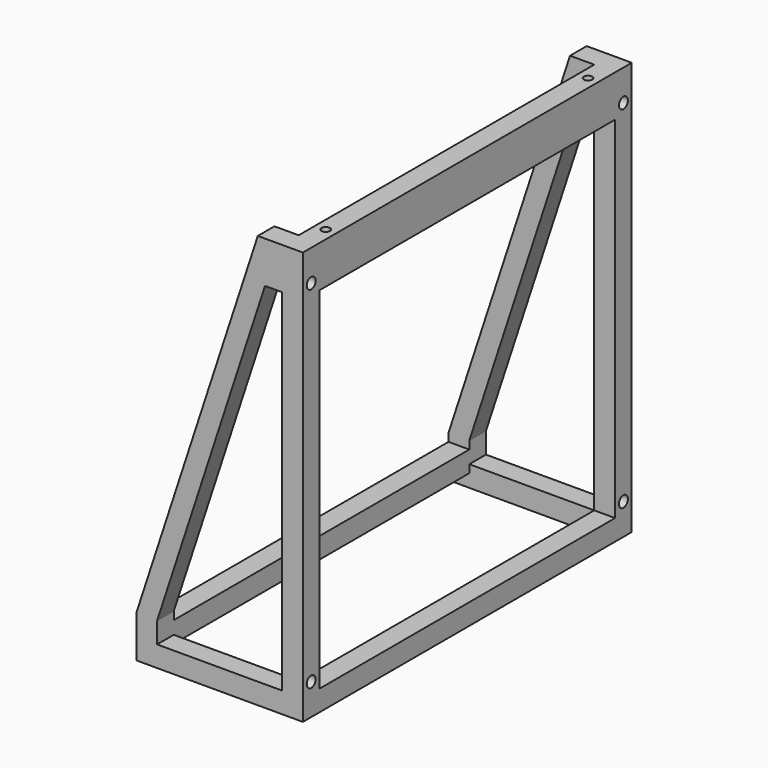
from build123d import *

# Parameters (mm, degrees)
F1_DEPTH = 12.7
F2_W     = 12.7
F2_H     = 12.7
F3_DEPTH = 225.300032
F4_W     = 12.7
F4_H     = 25.4
F5_DEPTH = 12.7
F7_D     = 6.8
F7_DEPTH = 15.75
F7_TIP   = 2.0429261047
F9_D     = 5.1054
F9_DEPTH = 16.51
F9_TIP   = 1.5338169022


# Not quite as in the source:
# - a feature names something its author has since deleted; it is built from what else it names


with BuildPart() as f1:
    # F0 (on Front) → F1 (new body)
    with BuildSketch(Plane.XZ):
        Polygon((0, 25.4), (0, 0), (101.6, 0), (101.6, 226.6), (101.6, 239.3), (101.6, 252), (74.1228589826, 252), align=None)
        Polygon((78.5142949131, 226.6), (88.9, 226.6), (88.9, 12.7), (12.7, 12.7), (12.7, 25.4), align=None, mode=Mode.SUBTRACT)
    extrude(amount=F1_DEPTH)

    # F2 (on face) → F3 (join)
    with BuildSketch(Plane(origin=(0, 0, 0), x_dir=(-1, 0, 0), z_dir=(0, 1, 0))):
        with Locations((-95.25, 6.35)):
            Rectangle(F2_W, F2_H)
        Polygon((-101.6, 252), (-101.6, 226.6), (-88.9, 226.6), (-88.9, 229.1588783264), (-88.9, 252), align=None)
        Polygon((-12.7, 20.574), (-12.7, 12.7), (-12.7, 7.874), (0, 7.874), (0, 20.574), align=None)
    extrude(amount=F3_DEPTH)

    # F4 (on face) → F5 (join)
    with BuildSketch(Plane(origin=(0, 225.300032, 0), x_dir=(-1, 0, 0), z_dir=(0, 1, 0))):
        Polygon((0, 0), (0, 25.4), (-74.1228589826, 252), (-88.9, 252), (-88.9, 226.6), (-101.6, 226.6), (-101.6, 0), align=None)
        Polygon((-88.9, 25.4), (-88.9, 226.6), (-78.5142949131, 226.6), (-12.7, 25.4), (-12.7, 12.7), (-88.9, 12.7), align=None, mode=Mode.SUBTRACT)
        with Locations((-95.25, 239.3)):
            Rectangle(F4_W, F4_H)
    extrude(amount=F5_DEPTH)

    # F7
    with Locations(Plane.YZ.offset(101.6)):
        with Locations((-6.35, 19), (-6.35, 233), (231.650032, 233), (231.650032, 19)):
            Hole(F7_D / 2, depth=F7_DEPTH)
            with Locations((0, 0, -(F7_DEPTH + F7_TIP / 2))):  # 118° drill point
                Cone(0, F7_D / 2, F7_TIP, mode=Mode.SUBTRACT)

    # F9
    with Locations(Plane.XY.offset(252)):
        with Locations((95.25, 212.600032), (95.25, 12.7)):
            Hole(F9_D / 2, depth=F9_DEPTH)
            with Locations((0, 0, -(F9_DEPTH + F9_TIP / 2))):  # 118° drill point
                Cone(0, F9_D / 2, F9_TIP, mode=Mode.SUBTRACT)


solid = f1.part
